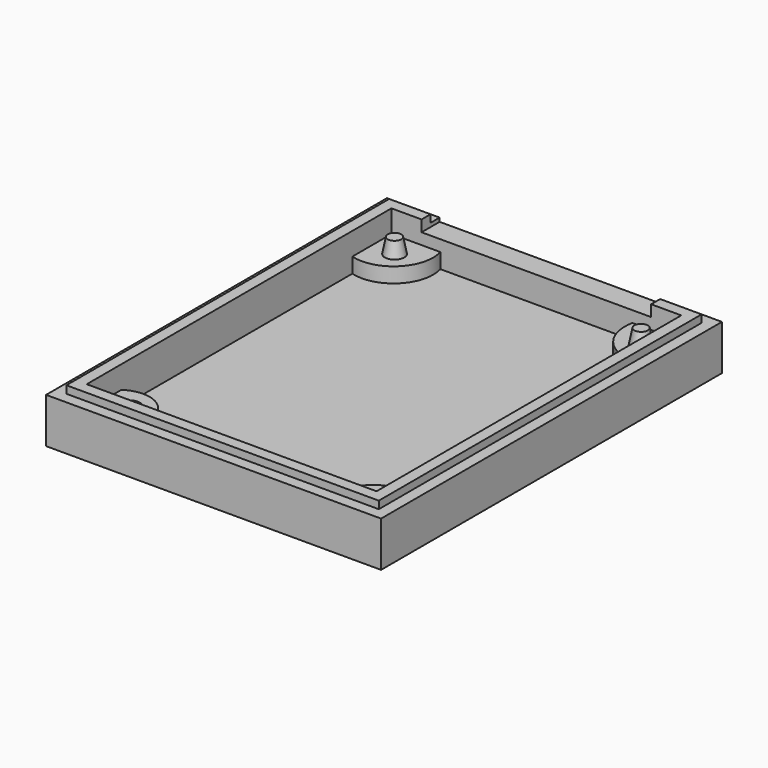
from build123d import *

# Parameters (mm, degrees)
F1_DEPTH = 2
F0_R     = 1.3
F0_R_2   = 1.5
F2_DEPTH = 4
F3_DEPTH = 6
F0_W     = 41.5
F0_H     = 53.6
F4_DEPTH = 7
F0_W_2   = 44.5
F0_H_2   = 56.6
F5_DEPTH = 6
F6_W     = 30.5
F6_H     = 1.5
F7_DEPTH = 3


# Not quite as in the source:
# - a fillet or chamfer that OpenCascade refuses, or shapes differently, is made with other operations: its cross-section is extruded or revolved along the edge and cut away or added
# - a feature names something its author has since deleted; it is built from what else it names


with BuildPart() as f1:
    # F0 (on Top) → F1 (new body)
    with BuildSketch(Plane.XY):
        with BuildLine():
            ThreePointArc((0, 5.75), (5.2603266711, 5.2603266711), (5.75, 0))
            Line((5.75, 0), (32.75, 0))
            ThreePointArc((32.75, 0), (33.3948928082, 5.1051071918), (38.5, 5.75))
            Line((38.5, 5.75), (38.5, 44.1))
            ThreePointArc((38.5, 44.1), (33.4963752154, 45.5963752154), (32, 50.6))
            Line((32, 50.6), (6.5, 50.6))
            ThreePointArc((6.5, 50.6), (5.1593928501, 45.4406071499), (0, 44.1))
            Line((0, 44.1), (0, 5.75))
        make_face()
    extrude(amount=F1_DEPTH)

    # F0 (on Top) → F2 (join)
    with BuildSketch(Plane.XY):
        with BuildLine():
            Line((0, 50.6), (0, 44.1))
            ThreePointArc((0, 44.1), (5.1593928501, 45.4406071499), (6.5, 50.6))
            Line((6.5, 50.6), (0, 50.6))
        make_face()
        with Locations((3.05, 47.3)):
            Circle(F0_R, mode=Mode.SUBTRACT)
        with BuildLine():
            ThreePointArc((32, 50.6), (33.4963752154, 45.5963752154), (38.5, 44.1))
            Line((38.5, 44.1), (38.5, 50.6))
            Line((38.5, 50.6), (32, 50.6))
        make_face()
        with Locations((35.8, 47.3)):
            Circle(F0_R, mode=Mode.SUBTRACT)
        with BuildLine():
            ThreePointArc((38.5, 5.75), (33.3948928082, 5.1051071918), (32.75, 0))
            Line((32.75, 0), (38.5, 0))
            Line((38.5, 0), (38.5, 5.75))
        make_face()
        with Locations((35.44, 2.9)):
            Circle(F0_R_2, mode=Mode.SUBTRACT)
        with BuildLine():
            Line((0, 5.75), (0, 0))
            Line((0, 0), (5.75, 0))
            ThreePointArc((5.75, 0), (5.2603266711, 5.2603266711), (0, 5.75))
        make_face()
        with Locations((3.01, 3.25)):
            Circle(F0_R_2, mode=Mode.SUBTRACT)
    extrude(amount=F2_DEPTH)

    # F0 (on Top) → F3 (join)
    with BuildSketch(Plane.XY):
        with Locations((3.05, 47.3)):
            Circle(F0_R)
        with Locations((35.8, 47.3)):
            Circle(F0_R)
    extrude(amount=F3_DEPTH)

    # F0 (on Top) → F4 (join)
    with BuildSketch(Plane.XY):
        with Locations((19.25, 25.3)):
            Rectangle(F0_W, F0_H)
        Polygon((5.75, 0), (0, 0), (0, 5.75), (0, 44.1), (0, 50.6), (6.5, 50.6), (32, 50.6), (38.5, 50.6), (38.5, 44.1), (38.5, 5.75), (38.5, 0), (32.75, 0), align=None, mode=Mode.SUBTRACT)
    extrude(amount=F4_DEPTH)

    # F0 (on Top) → F5 (join)
    with BuildSketch(Plane.XY):
        with Locations((19.25, 25.3)):
            Rectangle(F0_W_2, F0_H_2)
        with Locations((19.25, 25.3)):
            Rectangle(F0_W, F0_H, mode=Mode.SUBTRACT)
    extrude(amount=F5_DEPTH)

    # F6 (on face) → F7 (cut)
    with BuildSketch(Plane(origin=(0, 53.6, 0), x_dir=(-1, 0, 0), z_dir=(0, 1, 0))):
        with Locations((-19.25, 6.25)):
            Rectangle(F6_W, F6_H)
    extrude(amount=-F7_DEPTH, mode=Mode.SUBTRACT)

    # F8: chamfer of 0.4 x 2.0578216064 on 2 edges, made by hand


with BuildPart() as f8_tool2:
    # F8_s3 → F8_t4 (revolve)
    with BuildSketch(Plane.XZ.offset(-47.3)):
        Polygon((37.1, 3.9421783936), (36.7, 6), (37.1, 6), align=None)
    revolve(axis=Axis((35.8, 47.3, 6), (0, 0, 1)))

    split(bisect_by=Plane.XY.offset(4), keep=Keep.TOP)


with BuildPart() as f1_1:
    add(f1.part)

    # F8_t1: cut F8_tool2
    add(f8_tool2.part, mode=Mode.SUBTRACT)


with BuildPart() as f8_tool7:
    # F8_s8 → F8_t9 (revolve)
    with BuildSketch(Plane.XZ.offset(-47.3)):
        Polygon((4.35, 3.9421783936), (3.95, 6), (4.35, 6), align=None)
    revolve(axis=Axis((3.05, 47.3, 6), (0, 0, 1)))

    split(bisect_by=Plane.XY.offset(4), keep=Keep.TOP)


with BuildPart() as f1_2:
    add(f1_1.part)

    # F8_t6: cut F8_tool7
    add(f8_tool7.part, mode=Mode.SUBTRACT)


solid = f1_2.part
